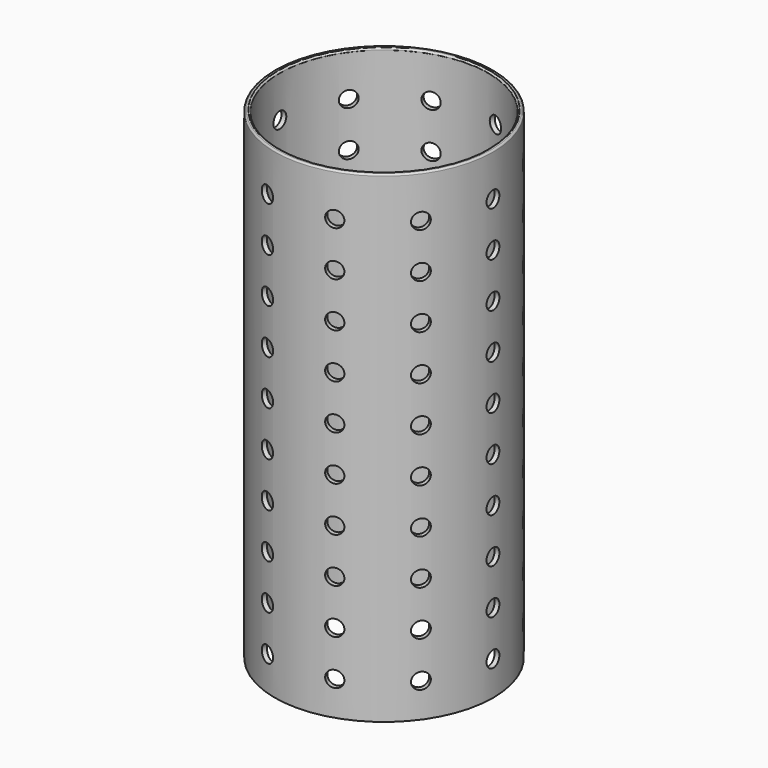
from build123d import *

# Parameters (mm, degrees)
F0_R            = 34
F0_R_2          = 32.5
F1_DEPTH        = 150
F3_R            = 2.5
F4_DEPTH        = 25
F4_COPIES_COUNT = 10
F5_R            = 0.5


# Not quite as in the source:
# - a pattern or mirror of a feature is missing from the dataset's text; its kind, count and spacing are read off the source's solid


with BuildPart() as f1:
    # F0 (on Top) → F1 (new body)
    with BuildSketch(Plane.XY):
        Circle(F0_R)
        Circle(F0_R_2, mode=Mode.SUBTRACT)
    extrude(amount=F1_DEPTH)

    # F3 (on offset) → F4 (cut)
    with BuildSketch(Plane.YZ.offset(50)):
        with Locations((0, 136.6552802026)):
            Circle(F3_R)
        with Locations((0, 122.6552802026)):
            Circle(F3_R)
        with Locations((0, 108.6552802026)):
            Circle(F3_R)
        with Locations((0, 94.6552802026)):
            Circle(F3_R)
        with Locations((0, 80.6552802026)):
            Circle(F3_R)
        with Locations((0, 66.6552802026)):
            Circle(F3_R)
        with Locations((0, 52.6552802026)):
            Circle(F3_R)
        with Locations((0, 38.6552802026)):
            Circle(F3_R)
        with Locations((0, 24.6552802026)):
            Circle(F3_R)
        with Locations((0, 10.6552802026)):
            Circle(F3_R)
    f4 = extrude(amount=-F4_DEPTH, mode=Mode.SUBTRACT)

    # F4_copies: F4 ×10 about axis
    f4_copies_axis = Axis((0, 0, 0), (0, 0, 1))
    for i in range(1, F4_COPIES_COUNT):
        add(f4.rotate(f4_copies_axis, i * 360 / F4_COPIES_COUNT), mode=Mode.SUBTRACT)

    # F5
    f5_edges = [f1.edges().sort_by_distance(p)[0] for p in [
        (-34, 0, 150),
        (-32.5, 0, 150),
    ]]
    fillet(f5_edges, radius=F5_R)


solid = f1.part
